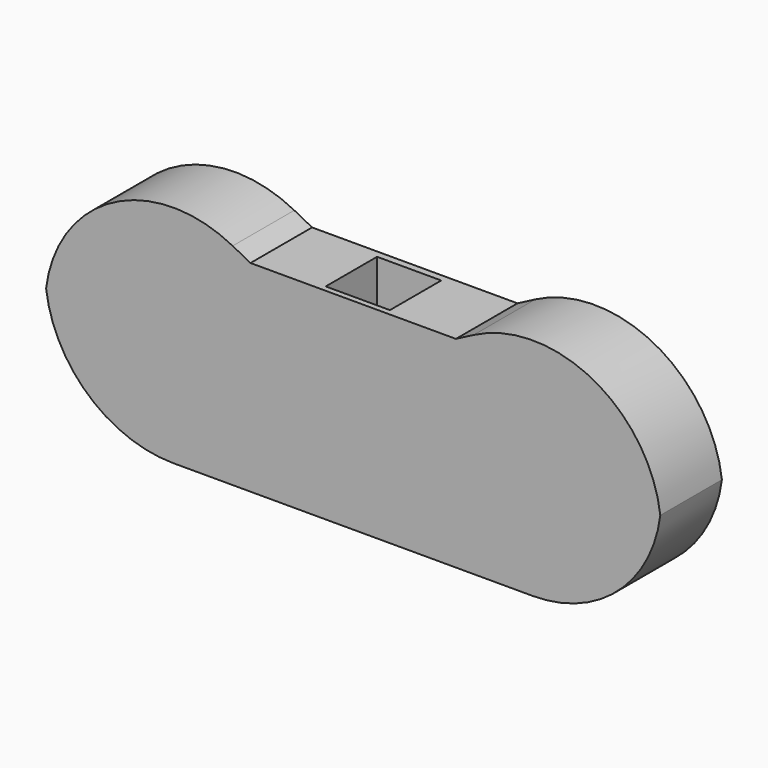
from build123d import *

# Parameters (mm, degrees)
F3_T1_DEPTH = 28
F3_T3_DEPTH = 44.1725614133
F5_W        = 2.5
F5_H        = 2.5


# Not quite as in the source:
# - a fillet or chamfer that OpenCascade refuses, or shapes differently, is made with other operations: its cross-section is extruded or revolved along the edge and cut away or added
# - two fillets or chamfers of one size are made in one step


with BuildPart() as f2:
    # F2: sweep along a path in F1
    with BuildLine(Plane.XY) as f2_path:
        Line((0, 0), (0, 3))
    # F0 (on Front) → F2 (sweep)
    with BuildSketch(Plane.XZ):
        Polygon((-12, 0), (0, 0), (12, 0), (12, 12), (4, 7.8411921859), (0, 7.8411921859), (-4, 7.8411921859), (-12, 12), align=None)
    sweep(path=f2_path.line)

    # F3: fillet of radius 5 on 4 edges, made by hand

    # F3_s2 → F3_t1 (cut)
    with BuildSketch(Plane.XZ.offset(-15.5)):
        with BuildLine():
            ThreePointArc((-7, 0), (-10.5355339059, 1.4644660941), (-12, 5))
            Line((-12, 5), (-12, 0))
            Line((-12, 0), (-7, 0))
        make_face()
        with BuildLine():
            ThreePointArc((7, 0), (10.5355339059, 1.4644660941), (12, 5))
            Line((12, 5), (12, 0))
            Line((12, 0), (7, 0))
        make_face()
    extrude(amount=F3_T1_DEPTH, mode=Mode.SUBTRACT)

    # F3_s4 → F3_t3 (cut)
    with BuildSketch(Plane.XZ.offset(-23.5862807066)):
        with BuildLine():
            ThreePointArc((-4.6937567356, 8.2018423025), (-9.5950706809, 8.0393159966), (-12, 3.7654877173))
            Line((-12, 3.7654877173), (-12, 12))
            Line((-12, 12), (-4.6937567356, 8.2018423025))
        make_face()
        with BuildLine():
            ThreePointArc((4.6937567356, 8.2018423025), (9.5950706809, 8.0393159966), (12, 3.7654877173))
            Line((12, 3.7654877173), (12, 12))
            Line((12, 12), (4.6937567356, 8.2018423025))
        make_face()
    extrude(amount=F3_T3_DEPTH, mode=Mode.SUBTRACT)

    # F7: sweep along a path in F6
    with BuildLine(Plane.XZ) as f7_path:
        Line((0, -1.2934210245), (0, 11.7065789755))
    # F5 (on Top) → F7 (sweep, cut)
    with BuildSketch(Plane.XY):
        with Locations((0, 1.4747590758)):
            Rectangle(F5_W, F5_H)
    sweep(path=f7_path.line, mode=Mode.SUBTRACT)


solid = f2.part
